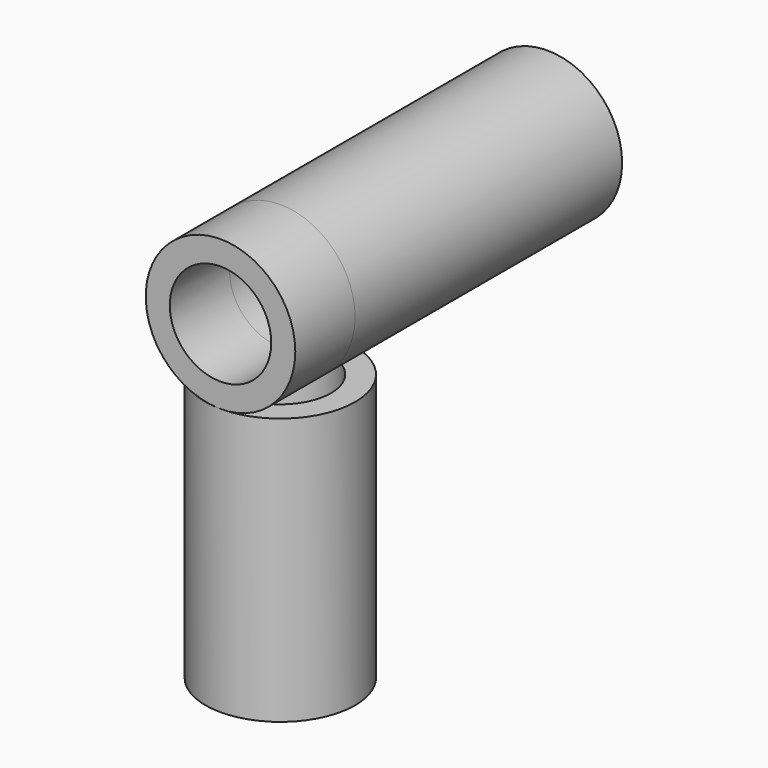
from build123d import *

# Parameters (mm, degrees)
F0_R          = 5.6
F0_R_2        = 3.8
F1_DEPTH      = 20
F2_R          = 5.6
F2_R_2        = 3.8
F3_DEPTH      = 25
F3_DEPTH_BACK = 5.6


with BuildPart() as f1:
    # F0 (on Top) → F1 (new body)
    with BuildSketch(Plane.XY):
        Circle(F0_R)
        Circle(F0_R_2, mode=Mode.SUBTRACT)
    extrude(amount=F1_DEPTH)


with BuildPart() as f3:
    # F2 (on Front) → F3 (new body, two sides)
    with BuildSketch(Plane.XZ) as f3_sk:
        with Locations((0, 25.6)):
            Circle(F2_R)
        with Locations((0, 25.6)):
            Circle(F2_R_2, mode=Mode.SUBTRACT)
    extrude(amount=-F3_DEPTH)
    extrude(f3_sk.sketch, amount=F3_DEPTH_BACK)


solid = Compound([f1.part, f3.part])
